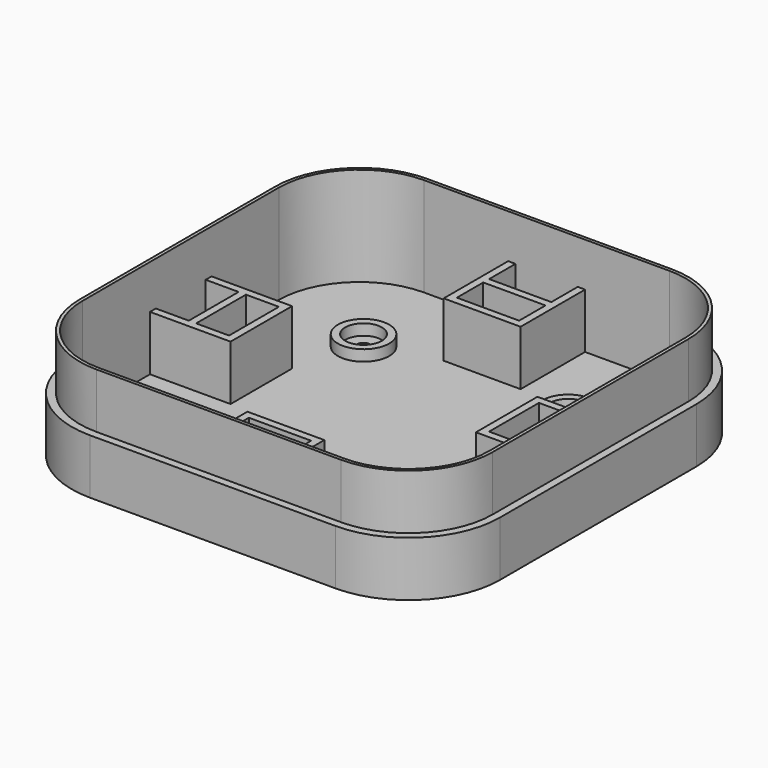
from build123d import *

# Parameters (mm, degrees)
F1_DEPTH      = 30
F2_T          = -3
F4_DEPTH      = 15
F5_R          = 1.75
F6_DEPTH      = 1
F7_R          = 7
F7_R_2        = 5
F8_DEPTH      = 3
F10_DEPTH     = 15
F11_W         = 2
F11_H         = 21
F11_W_2       = 21
F11_H_2       = 2
F12_DEPTH     = 15
F13_TEXT_SIZE = 9.7222222222
F14_DEPTH     = 1.5


# Not quite as in the source:
# - Text() gives the source's letters only with a copy of the font that has no kerning and outlines rounded to 1/6400 em; it was checked with that copy


with BuildPart() as f1:
    # F0 (on Top) → F1 (new body)
    with BuildSketch(Plane.XY):
        with BuildLine():
            ThreePointArc((58.5, 33.5), (51.1776695297, 51.1776695297), (33.5, 58.5))
            Line((33.5, 58.5), (-33.5, 58.5))
            ThreePointArc((-33.5, 58.5), (-51.1776695297, 51.1776695297), (-58.5, 33.5))
            Line((-58.5, 33.5), (-58.5, -33.5))
            ThreePointArc((-58.5, -33.5), (-51.1776695297, -51.1776695297), (-33.5, -58.5))
            Line((-33.5, -58.5), (33.5, -58.5))
            ThreePointArc((33.5, -58.5), (51.1776695297, -51.1776695297), (58.5, -33.5))
            Line((58.5, -33.5), (58.5, 33.5))
        make_face()
    extrude(amount=F1_DEPTH)

    # F2
    f2_openings = [f1.faces().sort_by_distance(p)[0] for p in [
        (0, 0, 30),
    ]]
    offset(amount=F2_T, openings=f2_openings)

    # F3 (on face) → F4 (cut)
    with BuildSketch(Plane.XY.offset(30)):
        with BuildLine():
            ThreePointArc((58.5, 33.5), (51.1776695297, 51.1776695297), (33.5, 58.5))
            Line((33.5, 58.5), (-33.5, 58.5))
            ThreePointArc((-33.5, 58.5), (-51.1776695297, 51.1776695297), (-58.5, 33.5))
            Line((-58.5, 33.5), (-58.5, -33.5))
            ThreePointArc((-58.5, -33.5), (-51.1776695297, -51.1776695297), (-33.5, -58.5))
            Line((-33.5, -58.5), (33.5, -58.5))
            ThreePointArc((33.5, -58.5), (51.1776695297, -51.1776695297), (58.5, -33.5))
            Line((58.5, -33.5), (58.5, 33.5))
        make_face()
        with BuildLine():
            Line((-33.4, 56.4), (33.4, 56.4))
            ThreePointArc((33.4, 56.4), (49.6634559673, 49.6634559673), (56.4, 33.4))
            Line((56.4, 33.4), (56.4, -33.4))
            ThreePointArc((56.4, -33.4), (49.6634559673, -49.6634559673), (33.4, -56.4))
            Line((33.4, -56.4), (-33.4, -56.4))
            ThreePointArc((-33.4, -56.4), (-49.6634559673, -49.6634559673), (-56.4, -33.4))
            Line((-56.4, -33.4), (-56.4, 33.4))
            ThreePointArc((-56.4, 33.4), (-49.6634559673, 49.6634559673), (-33.4, 56.4))
        make_face(mode=Mode.SUBTRACT)
    extrude(amount=-F4_DEPTH, mode=Mode.SUBTRACT)

    # F5 (on face) → F6 (cut)
    with BuildSketch(Plane.XY.offset(3)):
        with Locations((27.9307178569, 27.9307178569)):
            Circle(F5_R)
        with Locations((-27.9307178569, 27.9307178569)):
            Circle(F5_R)
        with Locations((27.9307178569, -27.9307178569)):
            Circle(F5_R)
        with Locations((-27.9307178569, -27.9307178569)):
            Circle(F5_R)
    extrude(amount=-F6_DEPTH, mode=Mode.SUBTRACT)

    # F7 (on face) → F8 (join)
    with BuildSketch(Plane.XY.offset(3)):
        with Locations((-27.9307178569, 27.9307178569)):
            Circle(F7_R)
        with Locations((-27.9307178569, 27.9307178569)):
            Circle(F7_R_2, mode=Mode.SUBTRACT)
        with Locations((27.9307178569, 27.9307178569)):
            Circle(F7_R)
        with Locations((27.9307178569, 27.9307178569)):
            Circle(F7_R_2, mode=Mode.SUBTRACT)
        with Locations((27.9307178569, -27.9307178569)):
            Circle(F7_R)
        with Locations((27.9307178569, -27.9307178569)):
            Circle(F7_R_2, mode=Mode.SUBTRACT)
        with Locations((-27.9307178569, -27.9307178569)):
            Circle(F7_R)
        with Locations((-27.9307178569, -27.9307178569)):
            Circle(F7_R_2, mode=Mode.SUBTRACT)
    extrude(amount=F8_DEPTH)

    # F9 (on face) → F10 (join)
    with BuildSketch(Plane.XY.offset(3)):
        Polygon((-8.5, 55.5), (-10.5, 55.5), (-10.5, 33.5), (10.5, 33.5), (10.5, 55.5), (8.5, 55.5), (8.5, 35.5), (-8.5, 35.5), align=None)
        Polygon((55.5, 8.5), (55.5, 10.5), (33.5, 10.5), (33.5, -10.5), (55.5, -10.5), (55.5, -8.5), (35.5, -8.5), (35.5, 8.5), align=None)
        Polygon((-10.5, -55.5), (-8.5, -55.5), (-8.5, -35.5), (8.5, -35.5), (8.5, -55.5), (10.5, -55.5), (10.5, -33.5), (-10.5, -33.5), align=None)
        Polygon((-33.5, 10.5), (-55.5, 10.5), (-55.5, 8.5), (-35.5, 8.5), (-35.5, -8.5), (-55.5, -8.5), (-55.5, -10.5), (-33.5, -10.5), align=None)
    extrude(amount=F10_DEPTH)

    # F11 (on face) → F12 (join)
    with BuildSketch(Plane.XY.offset(3)):
        with Locations((-45.5, 0)):
            Rectangle(F11_W, F11_H)
        with Locations((45.5, 0)):
            Rectangle(F11_W, F11_H)
        with Locations((0, -45.5)):
            Rectangle(F11_W_2, F11_H_2)
        with Locations((0, 45.5)):
            Rectangle(F11_W_2, F11_H_2)
    extrude(amount=F12_DEPTH)

    # F13 (on face) → F14 (cut)
    with BuildSketch(Plane(origin=(0, 0, 0), x_dir=(1, 0, 0), z_dir=(0, 0, -1))):
        with Locations((0, -32)):
            Text('Case by', F13_TEXT_SIZE, font='Tinos', font_style=FontStyle.ITALIC, text_align=(TextAlign.LEFT, TextAlign.BOTTOM))
        with Locations((0, -43.1805555556)):
            Text('PrototypeRC', F13_TEXT_SIZE, font='Tinos', font_style=FontStyle.ITALIC, text_align=(TextAlign.LEFT, TextAlign.BOTTOM))
    extrude(amount=-F14_DEPTH, mode=Mode.SUBTRACT)


solid = f1.part
